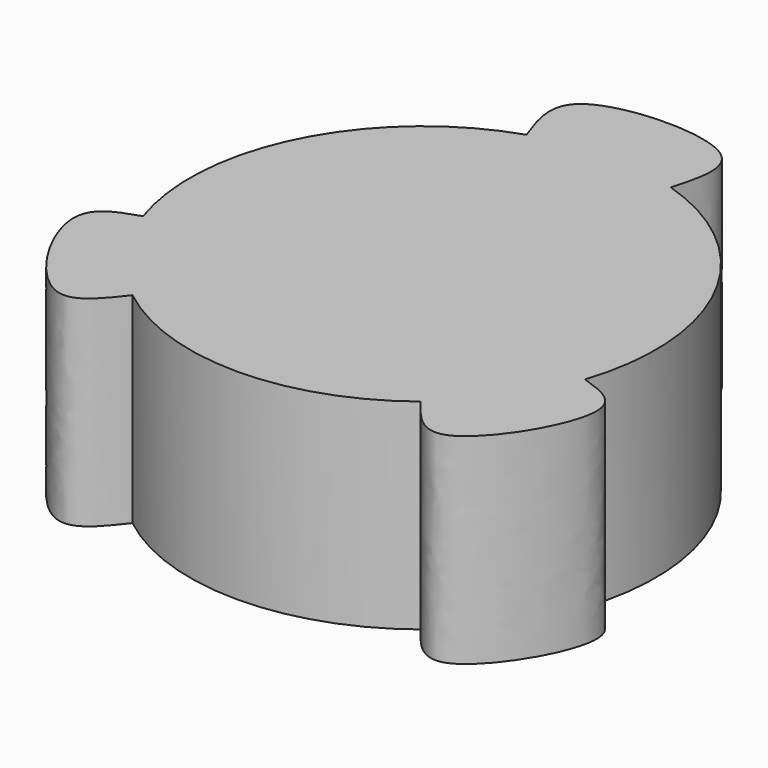
from build123d import *

# Parameters (mm, degrees)
F1_DEPTH = 50.8


with BuildPart() as f1:
    # F0 (on Top) → F1 (new body)
    with BuildSketch(Plane.XY):
        with BuildLine():
            add(Edge.make_bspline(
                [(-55.9372343089, -18.6110077969), (-60.8635430407, -20.2230194958), (-73.4053859661, -24.3510672229), (-49.5743515525, -63.3247808232), (-40.2484306998, -51.254227378), (-36.4546575654, -46.3292751415)],
                knots=[0, 0, 0, 0, 0.2757957407, 0.7062920031, 1, 1, 1, 1], degree=3))
            ThreePointArc((-36.4546575654, -46.3292751415), (0, -58.9520465577), (36.4546575654, -46.3292751415))
            add(Edge.make_bspline(
                [(55.9372343089, -18.6110077969), (60.8635430407, -20.2230194958), (73.4053859661, -24.3510672229), (49.5743515525, -63.3247808232), (40.2484306998, -51.254227378), (36.4546575654, -46.3292751415)],
                knots=[0, 0, 0, 0, 0.2757957407, 0.7062920031, 1, 1, 1, 1], degree=3))
            ThreePointArc((55.9372343089, -18.6110077969), (52.5276532647, 26.7617158615), (17.8266388345, 56.1921234801))
            add(Edge.make_bspline(
                [(-18.5308456371, 55.9638414811), (-20.8923301584, 62.4104470065), (-26.6259819502, 78.1207966464), (24.2945065208, 79.3302533373), (19.7307556094, 62.9747286546), (17.8266388345, 56.1921234801)],
                knots=[0, 0, 0, 0, 0.2886847661, 0.7062556792, 1, 1, 1, 1], degree=3))
            ThreePointArc((-18.5308456371, 55.9638414811), (-52.694646492, 26.4313833241), (-55.9372343089, -18.6110077969))
        make_face()
    extrude(amount=F1_DEPTH)


solid = f1.part
